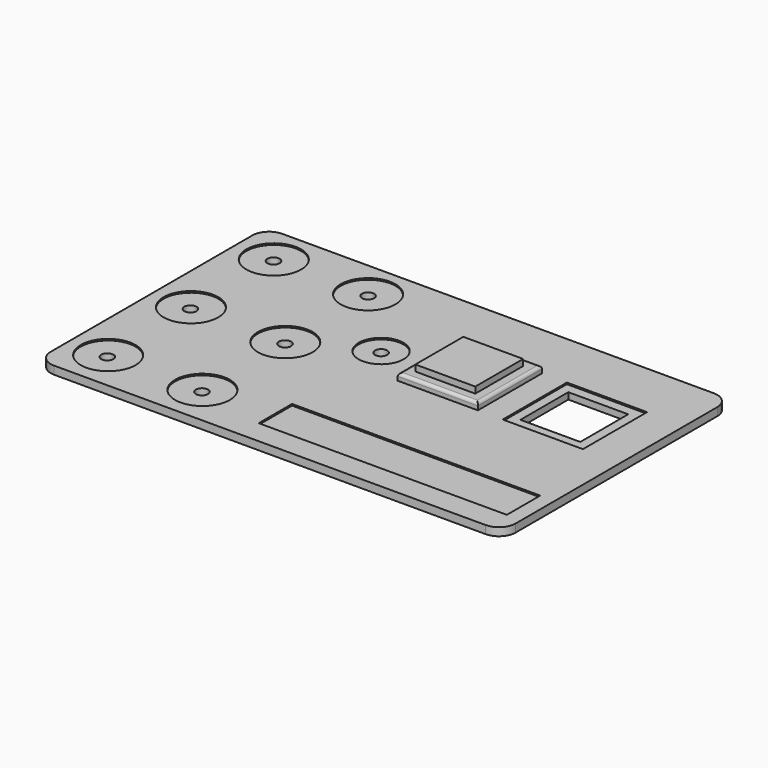
from build123d import *

# Parameters (mm, degrees)
F0_W     = 149.275535468
F0_H     = 88.9295647983
F0_R     = 9.2017219818
F0_W_2   = 83.4177359939
F0_H_2   = 14.016918838
F0_R_2   = 7.5380629756
F0_W_3   = 26.9511193037
F0_H_3   = 26.9511193037
F0_R_3   = 2.05
F0_W_4   = 20.125
F0_H_4   = 20.125
F1_DEPTH = 2.2
F2_DEPTH = 0.5
F3_DEPTH = 2.8
F4_R     = 1
F5_DEPTH = 4.9


with BuildPart() as f1:
    # F0 (on Top) → F1 (new body)
    with BuildSketch(Plane.XY):
        with BuildLine():
            Line((155.1135683298, -4.6552774664), (10.0380328618, -4.6552774664))
            ThreePointArc((10.0380328618, -4.6552774664), (6.0782348872, -6.2954794918), (4.4380328618, -10.2552774664))
            Line((4.4380328618, -10.2552774664), (4.4380328618, -94.9848422647))
            ThreePointArc((4.4380328618, -94.9848422647), (6.0782348872, -98.9446402393), (10.0380328618, -100.5848422647))
            Line((10.0380328618, -100.5848422647), (155.1135683298, -100.5848422647))
            ThreePointArc((155.1135683298, -100.5848422647), (159.0733663045, -98.9446402393), (160.7135683298, -94.9848422647))
            Line((160.7135683298, -94.9848422647), (160.7135683298, -10.2552774664))
            ThreePointArc((160.7135683298, -10.2552774664), (159.0733663045, -6.2954794918), (155.1135683298, -4.6552774664))
        make_face()
        with Locations((82.5758005958, -52.6200598655)):
            Rectangle(F0_W, F0_H, mode=Mode.SUBTRACT)
        with Locations((82.5758005958, -52.6200598655)):
            Rectangle(F0_W, F0_H)
        with Locations((17.3635222559, -87.018850666)):
            Circle(F0_R, mode=Mode.SUBTRACT)
        with Locations((49.0635222559, -87.018850666)):
            Circle(F0_R, mode=Mode.SUBTRACT)
        with Locations((114.1299642622, -85.567753762)):
            Rectangle(F0_W_2, F0_H_2, mode=Mode.SUBTRACT)
        with Locations((17.3635222559, -52.218850666)):
            Circle(F0_R, mode=Mode.SUBTRACT)
        with Locations((49.0635222559, -52.218850666)):
            Circle(F0_R, mode=Mode.SUBTRACT)
        with Locations((71.8833981295, -40.4814398784)):
            Circle(F0_R_2, mode=Mode.SUBTRACT)
        with Locations((17.3635222559, -17.418850666)):
            Circle(F0_R, mode=Mode.SUBTRACT)
        with Locations((49.0635222559, -17.418850666)):
            Circle(F0_R, mode=Mode.SUBTRACT)
        with Locations((99.3279069662, -37.4725610018)):
            Rectangle(F0_W_3, F0_H_3, mode=Mode.SUBTRACT)
        with Locations((134.6279069662, -37.4725610018)):
            Rectangle(F0_W_3, F0_H_3, mode=Mode.SUBTRACT)
        with Locations((17.3635222559, -17.418850666)):
            Circle(F0_R)
        with Locations((17.2635222559, -17.418850666)):
            Circle(F0_R_3, mode=Mode.SUBTRACT)
        with Locations((17.3635222559, -52.218850666)):
            Circle(F0_R)
        with Locations((17.2635222559, -52.318850666)):
            Circle(F0_R_3, mode=Mode.SUBTRACT)
        with Locations((17.3635222559, -87.018850666)):
            Circle(F0_R)
        with Locations((17.2635222559, -87.218850666)):
            Circle(F0_R_3, mode=Mode.SUBTRACT)
        with Locations((49.0635222559, -87.018850666)):
            Circle(F0_R)
        with Locations((49.0635222559, -87.218850666)):
            Circle(F0_R_3, mode=Mode.SUBTRACT)
        with Locations((49.0635222559, -52.218850666)):
            Circle(F0_R)
        with Locations((49.0635222559, -52.318850666)):
            Circle(F0_R_3, mode=Mode.SUBTRACT)
        with Locations((49.0635222559, -17.418850666)):
            Circle(F0_R)
        with Locations((49.0635222559, -17.418850666)):
            Circle(F0_R_3, mode=Mode.SUBTRACT)
        with Locations((71.8833981295, -40.4814398784)):
            Circle(F0_R_2)
        with Locations((71.8833981295, -40.4814398784)):
            Circle(F0_R_3, mode=Mode.SUBTRACT)
        with Locations((114.1299642622, -85.567753762)):
            Rectangle(F0_W_2, F0_H_2)
        with Locations((99.3279069662, -37.4725610018)):
            Rectangle(F0_W_3, F0_H_3)
        with Locations((99.0379891396, -37.3623677492)):
            Rectangle(F0_W_4, F0_H_4, mode=Mode.SUBTRACT)
        with Locations((134.6279069662, -37.4725610018)):
            Rectangle(F0_W_3, F0_H_3)
        with Locations((134.3379891396, -37.3623677492)):
            Rectangle(F0_W_4, F0_H_4, mode=Mode.SUBTRACT)
    extrude(amount=-F1_DEPTH)

    # F0 (on Top) → F2 (join)
    with BuildSketch(Plane.XY):
        with BuildLine():
            Line((155.1135683298, -4.6552774664), (10.0380328618, -4.6552774664))
            ThreePointArc((10.0380328618, -4.6552774664), (6.0782348872, -6.2954794918), (4.4380328618, -10.2552774664))
            Line((4.4380328618, -10.2552774664), (4.4380328618, -94.9848422647))
            ThreePointArc((4.4380328618, -94.9848422647), (6.0782348872, -98.9446402393), (10.0380328618, -100.5848422647))
            Line((10.0380328618, -100.5848422647), (155.1135683298, -100.5848422647))
            ThreePointArc((155.1135683298, -100.5848422647), (159.0733663045, -98.9446402393), (160.7135683298, -94.9848422647))
            Line((160.7135683298, -94.9848422647), (160.7135683298, -10.2552774664))
            ThreePointArc((160.7135683298, -10.2552774664), (159.0733663045, -6.2954794918), (155.1135683298, -4.6552774664))
        make_face()
        with Locations((82.5758005958, -52.6200598655)):
            Rectangle(F0_W, F0_H, mode=Mode.SUBTRACT)
        with Locations((82.5758005958, -52.6200598655)):
            Rectangle(F0_W, F0_H)
        with Locations((17.3635222559, -87.018850666)):
            Circle(F0_R, mode=Mode.SUBTRACT)
        with Locations((49.0635222559, -87.018850666)):
            Circle(F0_R, mode=Mode.SUBTRACT)
        with Locations((114.1299642622, -85.567753762)):
            Rectangle(F0_W_2, F0_H_2, mode=Mode.SUBTRACT)
        with Locations((17.3635222559, -52.218850666)):
            Circle(F0_R, mode=Mode.SUBTRACT)
        with Locations((49.0635222559, -52.218850666)):
            Circle(F0_R, mode=Mode.SUBTRACT)
        with Locations((71.8833981295, -40.4814398784)):
            Circle(F0_R_2, mode=Mode.SUBTRACT)
        with Locations((17.3635222559, -17.418850666)):
            Circle(F0_R, mode=Mode.SUBTRACT)
        with Locations((49.0635222559, -17.418850666)):
            Circle(F0_R, mode=Mode.SUBTRACT)
        with Locations((99.3279069662, -37.4725610018)):
            Rectangle(F0_W_3, F0_H_3, mode=Mode.SUBTRACT)
        with Locations((134.6279069662, -37.4725610018)):
            Rectangle(F0_W_3, F0_H_3, mode=Mode.SUBTRACT)
    extrude(amount=F2_DEPTH)


with BuildPart() as f3:
    # F0 (on Top) → F3 (new body)
    with BuildSketch(Plane.XY):
        with Locations((99.3279069662, -37.4725610018)):
            Rectangle(F0_W_3, F0_H_3)
        with Locations((99.0379891396, -37.3623677492)):
            Rectangle(F0_W_4, F0_H_4, mode=Mode.SUBTRACT)
    extrude(amount=F3_DEPTH)

    # F4
    f4_edges = [f3.edges().sort_by_distance(p)[0] for p in [
        (99.327907, -50.948121, 2.8),
        (85.852347, -37.472561, 2.8),
        (99.327907, -23.997001, 2.8),
        (112.803467, -37.472561, 2.8),
    ]]
    fillet(f4_edges, radius=F4_R)

    # F0 (on Top) → F5 (join)
    with BuildSketch(Plane.XY):
        with Locations((99.0379891396, -37.3623677492)):
            Rectangle(F0_W_4, F0_H_4)
    extrude(amount=F5_DEPTH)


solid = Compound([f1.part, f3.part])
